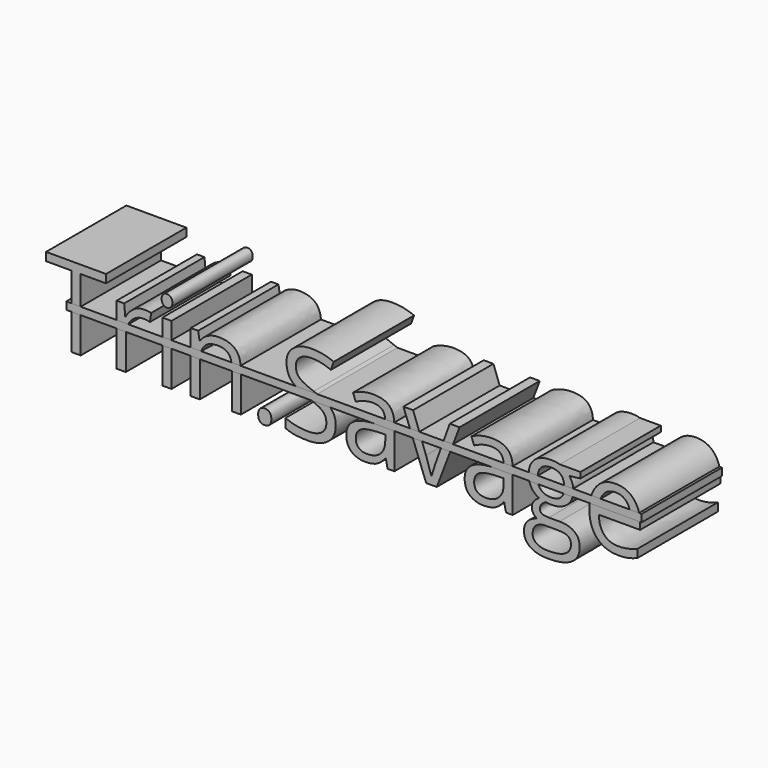
from build123d import *

# Parameters (mm, degrees)
F0_TEXT_SIZE = 28.3386600035
F1_DEPTH     = 25.4
F2_W         = 145.5737799406
F2_H         = 1.8816739321
F3_DEPTH     = 25.4


# Not quite as in the source:
# - Text() gives the source's letters only with a copy of the font that has no kerning and outlines rounded to 1/6400 em; it was checked with that copy


with BuildPart() as f1:
    # F0 (on Front) → F1 (new body)
    with BuildSketch(Plane.XZ):
        with Locations((-5.3694312178, -34.9012986342)):
            Text('Trin.Savage', F0_TEXT_SIZE, font='Open Sans', text_align=(TextAlign.LEFT, TextAlign.BOTTOM))
    extrude(amount=F1_DEPTH)


with BuildPart() as f3:
    # F2 (on Front) → F3 (new body)
    with BuildSketch(Plane.XZ):
        with Locations((72.7868899703, -24.9859411269)):
            Rectangle(F2_W, F2_H)
    extrude(amount=F3_DEPTH)


solid = Compound([f1.part, f3.part])
